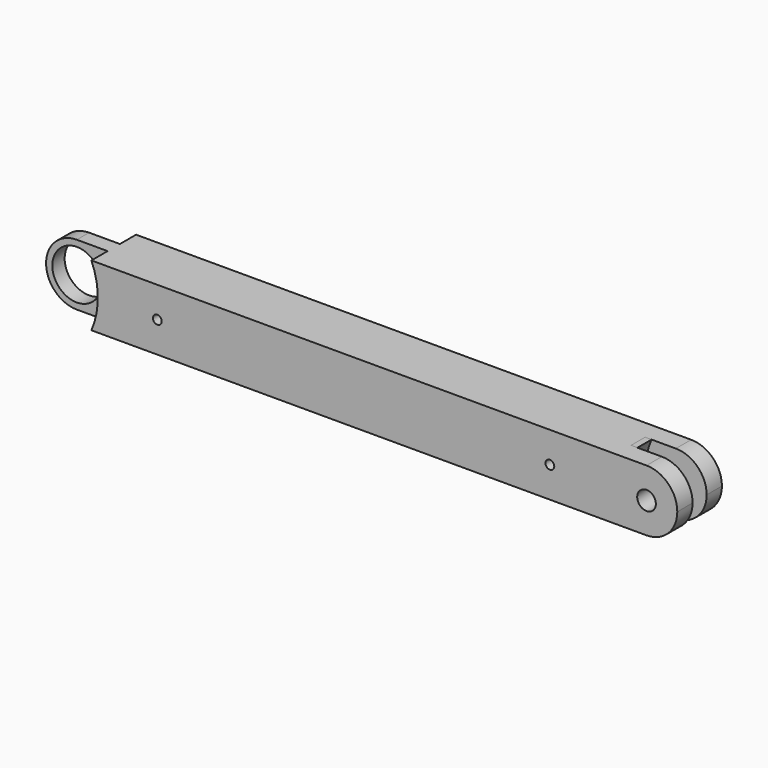
from build123d import *

# Parameters (mm, degrees)
F2_DEPTH  = 28
F3_DEPTH  = 28
F4_DEPTH  = 28
F5_R      = 11.15
F6_DEPTH  = 16.2
F5_R_2    = 4.25
F7_DEPTH  = 25.4
F8_DEPTH  = 16.7
F9_DEPTH  = 9.2
F12_R     = 2
F13_DEPTH = 25.4


with BuildPart() as f2:
    # F1 (on Top) → F2 (new body)
    with BuildSketch(Plane.XY):
        Polygon((-88.35, 12.7), (-133.35, 12.7), (-133.35, 3.5), (-161.35, 3.5), (-161.35, -3.5), (-133.35, -3.5), (-133.35, -12.7), (-118.35, -12.7), (-118.35, 0), (-88.35, 0), align=None)
    extrude(amount=F2_DEPTH)

    # F5 (on face) → F6 (cut, through all)
    with BuildSketch(Plane.XZ.offset(12.7)):
        with Locations((-147.35, 14)):
            Circle(F5_R)
        with BuildLine():
            Line((-161.35, 28), (-161.35, 14))
            ThreePointArc((-161.35, 14), (-157.2494949366, 23.8994949366), (-147.35, 28))
            Line((-147.35, 28), (-161.35, 28))
        make_face()
        with BuildLine():
            Line((-161.35, 14), (-161.35, 0))
            Line((-161.35, 0), (-147.35, 0))
            ThreePointArc((-147.35, 0), (-157.2494949366, 4.1005050634), (-161.35, 14))
        make_face()
    extrude(amount=-F6_DEPTH, mode=Mode.SUBTRACT)



with BuildPart() as f3:
    # F1 (on Top) → F3 (new body, through all)
    with BuildSketch(Plane.XY):
        Polygon((60.35, 12.7), (-88.35, 12.7), (-88.35, 0), (-118.35, 0), (-118.35, -12.7), (90.35, -12.7), (90.35, 0), (60.35, 0), align=None)
    extrude(amount=F3_DEPTH)


with BuildPart() as f4:
    # F1 (on Top) → F4 (new body, through all)
    with BuildSketch(Plane.XY):
        Polygon((133.35, 12.7), (60.35, 12.7), (60.35, 0), (90.35, 0), (90.35, -12.7), (133.35, -12.7), (133.35, -4), (105.35, -4), (105.35, 4), (133.35, 4), align=None)
    extrude(amount=F4_DEPTH)

    # F5 (on face) → F7 (cut, through all)
    with BuildSketch(Plane.XZ.offset(12.7)):
        with Locations((119.35, 14)):
            Circle(F5_R_2)
        with BuildLine():
            Line((133.35, 28), (119.35, 28.0000000002))
            ThreePointArc((119.35, 28.0000000001), (129.2494949366, 23.8994949367), (133.35, 14.0000000001))
            Line((133.35, 14.0000000001), (133.35, 28))
        make_face()
        with BuildLine():
            ThreePointArc((133.35, 14.0000000001), (129.2494949366, 4.1005050634), (119.35, 0))
            Line((119.35, 0), (133.35, 0))
            Line((133.35, 1e-10), (133.35, 14.0000000001))
        make_face()
    extrude(amount=-F7_DEPTH, mode=Mode.SUBTRACT)


with BuildPart() as f2_1:
    add(f2.part)

    add(f3.part)  # F8 merges F3

    add(f4.part)  # F8 merges F4
    # F5 (on face) → F8 (join, through all)
    with BuildSketch(Plane.XZ.offset(12.7)):
        with BuildLine():
            Line((105.35, 28.0000000004), (105.35, 14.0000000001))
            ThreePointArc((105.35, 14.0000000001), (106.0882790475, 21.1508375293), (108.2719701354, 28.0000000003))
            Line((108.2719701354, 28.0000000003), (105.35, 28.0000000004))
        make_face()
        with BuildLine():
            Line((105.35, 14.0000000001), (105.35, 2e-10))
            Line((105.35, 0), (108.2719701353, 0))
            ThreePointArc((108.2719701353, 0), (106.0882790474, 6.8491624709), (105.35, 14.0000000001))
        make_face()
    extrude(amount=-F8_DEPTH)

    # F10: F9 across plane


with BuildPart() as f9:
    # F5 (on face) → F9 (new body, through all)
    with BuildSketch(Plane.XZ.offset(12.7)):
        with BuildLine():
            Line((-133.35, 28), (-133.35, 0))
            ThreePointArc((-133.35, 0), (-130.4280298647, 14), (-133.35, 28))
        make_face()
    extrude(amount=-F9_DEPTH)


with BuildPart() as f2_2:
    add(f2_1.part)
    add(f9.part.mirror(Plane.XZ), mode=Mode.SUBTRACT)

    # F11: cut F9
    add(f9.part, mode=Mode.SUBTRACT)

    # F12 (on face) → F13 (cut, through all)
    with BuildSketch(Plane.XZ.offset(12.7)):
        with Locations((-103.35, 14)):
            Circle(F12_R)
        with Locations((75.35, 14.0000000006)):
            Circle(F12_R)
    extrude(amount=-F13_DEPTH, mode=Mode.SUBTRACT)


solid = f2_2.part
